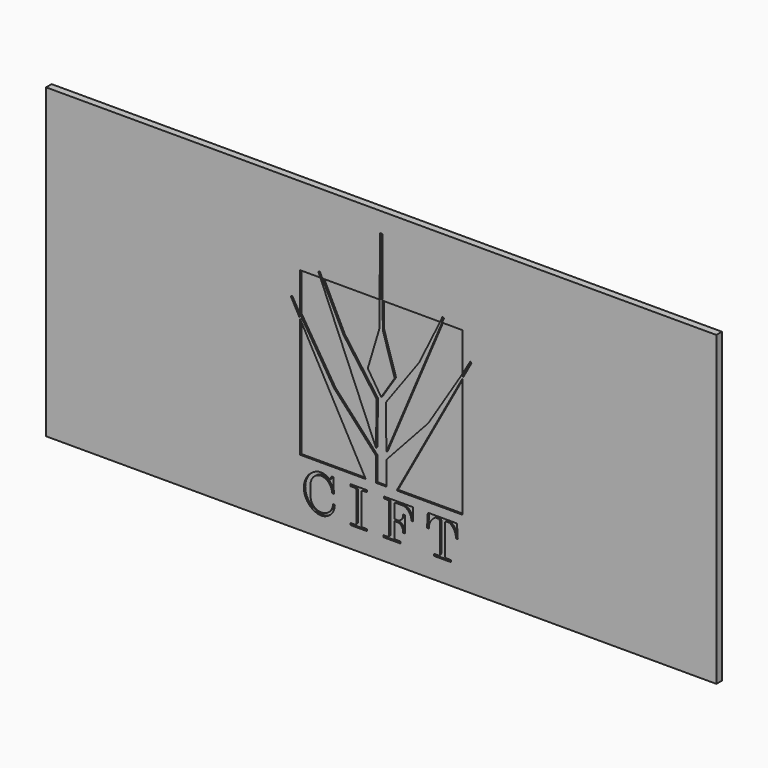
from build123d import *

# Parameters (mm, degrees)
F0_W     = 1219.2
F0_H     = 558.8
F1_DEPTH = 12.7
F3_DEPTH = 3.175


# Not quite as in the source:
# - ends of sketch curves that miss each other by under 0.0002 mm in the source are joined


with BuildPart() as f1:
    # F0 (on Front) → F1 (new body)
    with BuildSketch(Plane.XZ):
        Rectangle(F0_W, F0_H)
    extrude(amount=F1_DEPTH)

    # F2 (on face) → F3 (cut)
    with BuildSketch(Plane.XZ.offset(12.7)):
        Polygon((-110.776385, 136.9130104), (-147.738846, 136.9130104), (-147.738846, 66.8081214), (-85.6601792, -32.312991), (-9.521317, -115.3251186), (-9.521317, -158.7848488), (9.521317, -158.7848488), (9.521317, -115.3251186), (85.6601538, -32.312991), (147.738846, 66.8081214), (147.738846, 136.9130104), (110.7763596, 136.9130104), (9.470136, -102.9111988), (8.4179664, -24.1473228), (68.9105556, 59.2761832), (107.1551832, 136.9130104), (2.6089356, 136.9130104), (2.900426, 89.6063994), (24.4521482, 19.6980556), (-0.0642366, -18.3666638), (-24.4521482, 19.6980556), (-3.439668, 89.6063994), (-3.0142434, 136.9130104), (-107.1551832, 136.9130104), (-68.9105556, 59.2761832), (-8.4179918, -24.1473228), (-9.470136, -102.9111988), align=None)
        Polygon((-28.2203906, -158.7848488), (-147.738846, 59.252739), (-147.738846, -158.7848488), align=None)
        Polygon((147.738846, -158.7848488), (147.738846, 59.252739), (28.2203652, -158.7848488), align=None)
        with BuildLine():
            ThreePointArc((-109.8671422064, -179.8267368126), (-95.356903919, -186.4744799885), (-89.4000786424, -201.2817666107))
            Line((-89.4000786424, -201.2817666107), (-86.0775266, -201.2817666))
            Line((-86.0775266, -201.2817666), (-87.228807, -174.6107506))
            Line((-87.228807, -174.6107506), (-90.1839446, -174.6107506))
            Line((-90.1839446, -174.6107506), (-93.0793668, -180.8493462))
            ThreePointArc((-93.0793668, -180.8493462), (-102.7053794925, -175.5791240788), (-113.6444505241, -174.7004700875))
            ThreePointArc((-113.6444505241, -174.7004700875), (-140.7442467729, -209.1274434593), (-113.39827807, -243.3592184707))
            ThreePointArc((-113.39827807, -243.3592184707), (-93.1382802166, -237.533313942), (-84.4416180716, -218.3297640292))
            Line((-84.4416180716, -218.3297640292), (-87.6078766, -218.329764))
            ThreePointArc((-87.6078766, -218.329764), (-93.9825550775, -232.5723606205), (-108.5038975848, -238.2836063253))
            ThreePointArc((-108.5038975848, -238.2836063253), (-122.8229554836, -232.9071157052), (-128.4500788749, -218.68467849))
            Line((-128.4500788749, -218.68467849), (-128.450086, -203.0753622))
            ThreePointArc((-128.450086, -203.0753622), (-124.1111022303, -187.4924501184), (-109.8671422064, -179.8267368126))
        make_face()
        with BuildLine():
            Line((-55.665624, -238.077629), (-55.665624, -241.4936496))
            Line((-55.665624, -241.4936496), (-25.422352, -241.4936496))
            Line((-25.422352, -241.4936496), (-25.422352, -238.077629))
            Line((-25.422352, -238.077629), (-32.919924, -238.077629))
            ThreePointArc((-32.919924, -238.077629), (-35.0246805086, -237.2058103086), (-35.8964992, -235.1010538))
            Line((-35.8964992, -235.1010538), (-35.8964738, -182.243603))
            ThreePointArc((-35.8964738, -182.243603), (-35.0246805086, -180.1388464914), (-32.919924, -179.2670278))
            Line((-32.919924, -179.2670278), (-25.422352, -179.2670532))
            Line((-25.422352, -179.2670532), (-25.422352, -175.8510072))
            Line((-25.422352, -175.8510072), (-55.665624, -175.8510072))
            Line((-55.665624, -175.8510072), (-55.665624, -179.2670532))
            Line((-55.665624, -179.2670532), (-48.0573588, -179.2670532))
            ThreePointArc((-48.0573588, -179.2670532), (-45.9526022914, -180.1388464914), (-45.0807836, -182.243603))
            Line((-45.0807836, -182.243603), (-45.080809, -235.1010538))
            ThreePointArc((-45.080809, -235.1010538), (-45.9526022914, -237.2058103086), (-48.0573588, -238.077629))
            Line((-48.0573588, -238.077629), (-55.665624, -238.077629))
        make_face()
        with BuildLine():
            Line((31.9159128, -205.8210006), (23.7701836, -205.8210006))
            Line((23.7701836, -205.8210006), (23.7701836, -182.2325286))
            ThreePointArc((23.7701836, -182.2325286), (24.6423974564, -180.1274129149), (26.7478255999, -179.2559789912))
            Line((26.7478255999, -179.2559789912), (41.0262324, -179.2611096))
            ThreePointArc((41.0262324, -179.2611096), (51.1481998687, -186.6406443843), (55.0079383919, -198.557616598))
            Line((55.0079383919, -198.557616598), (58.1934574, -198.5576166))
            Line((58.1934574, -198.5576166), (57.3842134, -175.8510072))
            Line((57.3842134, -175.8510072), (5.1603656, -175.8321858))
            Line((5.1603656, -175.8321858), (5.153533, -179.2482064))
            Line((5.153533, -179.2482064), (11.6103908, -179.2505178))
            ThreePointArc((11.6103908, -179.2505178), (13.7144412242, -180.1227226778), (14.5858738, -182.227093))
            Line((14.5858738, -182.227093), (14.5858738, -235.1010538))
            ThreePointArc((14.5858738, -235.1010538), (13.7140551086, -237.2058103086), (11.6092986, -238.077629))
            Line((11.6092986, -238.077629), (3.801745, -238.077629))
            Line((3.801745, -238.077629), (3.801745, -241.4936496))
            Line((3.801745, -241.4936496), (35.4731574, -241.4936496))
            Line((35.4731574, -241.4936496), (35.4731574, -238.077629))
            Line((35.4731574, -238.077629), (26.7467588, -238.077629))
            ThreePointArc((26.7467588, -238.077629), (24.6420022914, -237.2058103086), (23.7701836, -235.1010538))
            Line((23.7701836, -235.1010538), (23.7701836, -209.2370212))
            Line((23.7701836, -209.2370212), (31.9159128, -209.2370212))
            ThreePointArc((31.9159128, -209.2370212), (37.6830347812, -213.8514597759), (39.8617861947, -220.9087784101))
            Line((39.8617861947, -220.9087784101), (39.8617948, -222.7084954))
            Line((39.8617948, -222.7084954), (43.1732436, -222.7084954))
            Line((43.1732436, -222.7084954), (43.1732436, -193.1940002))
            Line((43.1732436, -193.1940002), (39.8617948, -193.1940002))
            Line((39.8617948, -193.1940002), (39.8617948, -194.1492434))
            ThreePointArc((39.8617948, -194.1492434), (37.6830347812, -201.2065620241), (31.9159128, -205.8210006))
        make_face()
        with BuildLine():
            Line((106.7346608, -182.243603), (106.7346608, -235.1010538))
            ThreePointArc((106.7346608, -235.1010538), (105.8628421086, -237.2058103086), (103.7580856, -238.077629))
            Line((103.7580856, -238.077629), (96.1487536, -238.077629))
            Line((96.1487536, -238.077629), (96.1487536, -241.4936496))
            Line((96.1487536, -241.4936496), (126.6514358, -241.4936496))
            Line((126.6514358, -241.4936496), (126.6514358, -238.077629))
            Line((126.6514358, -238.077629), (118.8955458, -238.077629))
            ThreePointArc((118.8955458, -238.077629), (116.7907892914, -237.2058103086), (115.9189706, -235.1010538))
            Line((115.9189706, -235.1010538), (115.9189706, -182.243603))
            ThreePointArc((115.9189706, -182.243603), (116.7907892914, -180.1388464914), (118.8955458, -179.2670278))
            Line((118.8955458, -179.2670278), (124.14758, -179.2670532))
            ThreePointArc((124.14758, -179.2670532), (132.9675370035, -188.3940946035), (135.9963466509, -200.7197153285))
            Line((135.9963466509, -200.7197153285), (139.3194572, -200.7197154))
            Line((139.3194572, -200.7197154), (137.8614718, -175.8510072))
            Line((137.8614718, -175.8510072), (84.7921596, -175.8510072))
            Line((84.7921596, -175.8510072), (83.3341742, -200.7197154))
            Line((83.3341742, -200.7197154), (86.6572816, -200.7197154))
            ThreePointArc((86.6572816, -200.7197154), (89.6860943965, -188.3940946035), (98.5060445889, -179.2670418075))
            Line((98.5060445889, -179.2670418075), (103.7580856, -179.2670532))
            ThreePointArc((103.7580856, -179.2670532), (105.8628421086, -180.1388464914), (106.7346608, -182.243603))
        make_face()
        Polygon((-2.0544028, 243.6519638), (-2.9994959967, 138.552993536), (2.5988306881, 138.552993536), (1.9512534, 243.6519638), align=None)
        Polygon((-164.3414798, 89.5408928), (-148.8750427961, 61.3255006909), (-148.8750427961, 68.7675664065), (-161.7813884, 91.0253958), align=None)
        Polygon((-111.3482406, 146.2952116), (-114.2778258, 145.2020718), (-111.0982667862, 137.6750104), (-107.4957333194, 137.6750104), align=None)
        Polygon((111.0982437212, 137.6750104), (114.2778258, 145.2020718), (111.3482406, 146.2952116), (107.4957333194, 137.6750104), align=None)
        Polygon((164.3414798, 89.5408928), (161.7813884, 91.0253958), (148.5202014446, 68.1556195002), (148.5202014446, 60.6781642768), align=None)
    extrude(amount=-F3_DEPTH, mode=Mode.SUBTRACT)


solid = f1.part
